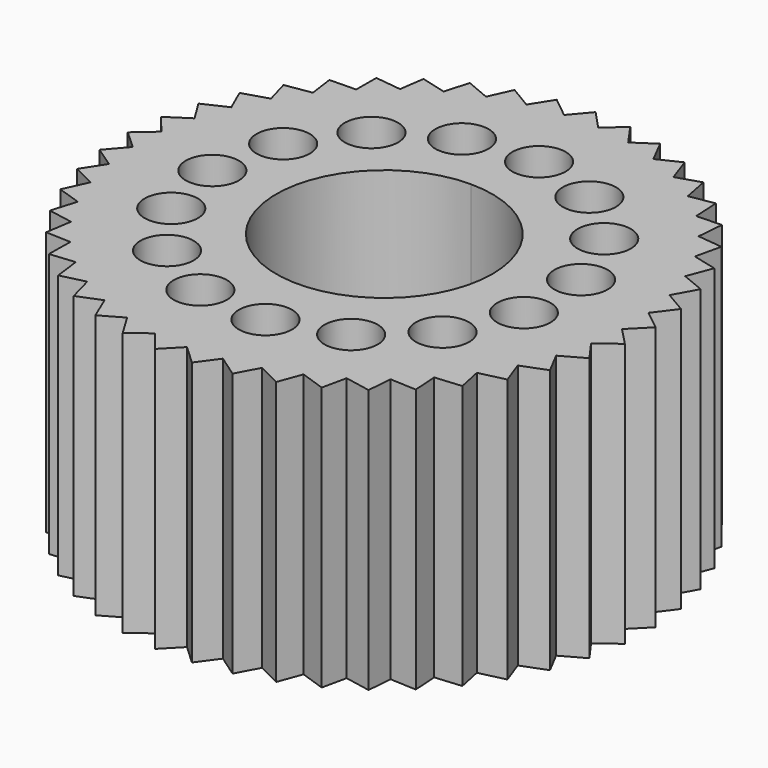
from build123d import *

# Parameters (mm, degrees)
F0_R            = 25.4
F1_DEPTH        = 25.4
F3_DEPTH        = 25.4
F6_DEPTH        = 25.4
F5_DEPTH        = 25.4
F5_COPIES_COUNT = 15


# Not quite as in the source:
# - a pattern or mirror of a feature is missing from the dataset's text; its kind, count and spacing are read off the source's solid


with BuildPart() as f1:
    # F0 (on Top) → F1 (new body)
    with BuildSketch(Plane.XY):
        Circle(F0_R)
    extrude(amount=F1_DEPTH)

    # F2 (on face) → F3 (cut)
    with BuildSketch(Plane.XY.offset(25.4)):
        with BuildLine():
            Line((-3.3733606068, -23.3670165801), (-5.2809569468, -24.8449490586))
            ThreePointArc((-5.2809569468, -24.8449490586), (-3.5349967644, -25.152808946), (-1.7718144331, -25.3381268766))
            Line((-1.7718144331, -25.3381268766), (-3.3733606068, -23.3670165801))
        make_face()
        with BuildLine():
            Line((-0.0884711356, -23.6090914373), (-1.7718144331, -25.3381268766))
            ThreePointArc((-1.7718144331, -25.3381268766), (0, -25.4), (1.7718144331, -25.3381268766))
            Line((1.7718144331, -25.3381268766), (-0.0884711356, -23.6090914373))
        make_face()
        with BuildLine():
            ThreePointArc((1.7718144331, -25.3381268766), (3.5349967644, -25.152808946), (5.2809569468, -24.8449490586))
            Line((5.2809569468, -24.8449490586), (3.1981403256, -23.3916421847))
            Line((3.1981403256, -23.3916421847), (1.7718144331, -25.3381268766))
        make_face()
        with BuildLine():
            ThreePointArc((5.2809569468, -24.8449490586), (7.0011888378, -24.4160470768), (8.6873116405, -23.868192568))
            Line((8.6873116405, -23.868192568), (6.4225036232, -22.7189012245))
            Line((6.4225036232, -22.7189012245), (5.2809569468, -24.8449490586))
        make_face()
        with BuildLine():
            ThreePointArc((8.6873116405, -23.868192568), (10.3311107341, -23.2040546241), (11.9245776948, -22.4268688586))
            Line((11.9245776948, -22.4268688586), (9.5218601932, -21.6039626944))
            Line((9.5218601932, -21.6039626944), (8.6873116405, -23.868192568))
        make_face()
        with BuildLine():
            ThreePointArc((11.9245776948, -22.4268688586), (13.4599493115, -21.5404216424), (14.9297454082, -20.5490316571))
            Line((14.9297454082, -20.5490316571), (12.4358845856, -20.0685276045))
            Line((12.4358845856, -20.0685276045), (11.9245776948, -22.4268688586))
        make_face()
        with BuildLine():
            ThreePointArc((14.9297454082, -20.5490316571), (16.326805286, -19.4575288552), (17.6443226097, -18.2712309286))
            Line((17.6443226097, -18.2712309286), (15.1078586301, -18.1424814524))
            Line((15.1078586301, -18.1424814524), (14.9297454082, -20.5490316571))
        make_face()
        with BuildLine():
            ThreePointArc((17.6443226097, -18.2712309286), (18.8758785671, -16.9959174015), (20.0154731416, -15.6378014733))
            Line((20.0154731416, -15.6378014733), (17.4857753913, -15.8633125357))
            Line((17.4857753913, -15.8633125357), (17.6443226097, -18.2712309286))
        make_face()
        with BuildLine():
            ThreePointArc((20.0154731416, -15.6378014733), (21.0575543429, -14.2034997482), (21.9970452561, -12.7))
            Line((21.9970452561, -12.7), (19.5233514242, -13.2753822847))
            Line((19.5233514242, -13.2753822847), (20.0154731416, -15.6378014733))
        make_face()
        with BuildLine():
            ThreePointArc((21.9970452561, -12.7), (22.829368776, -11.1346271284), (23.550469906, -9.5150074728))
            Line((23.550469906, -9.5150074728), (21.1809276292, -10.429061818))
            Line((21.1809276292, -10.429061818), (21.9970452561, -12.7))
        make_face()
        with BuildLine():
            ThreePointArc((23.550469906, -9.5150074728), (24.1568355139, -7.8490316571), (24.6455114474, -6.1448161482))
            Line((24.6455114474, -6.1448161482), (22.4262411709, -7.3797515259))
            Line((22.4262411709, -7.3797515259), (23.550469906, -9.5150074728))
        make_face()
        with BuildLine():
            ThreePointArc((24.6455114474, -6.1448161482), (25.0141169265, -4.4106637127), (25.2608561424, -2.655022967))
            Line((25.2608561424, -2.655022967), (23.2350534376, -4.1868027647))
            Line((23.2350534376, -4.1868027647), (24.6455114474, -6.1448161482))
        make_face()
        with BuildLine():
            ThreePointArc((25.4, 0), (25.396131457, 0.4432911235), (25.3845270063, 0.8864472162))
            Line((25.3845270063, 0.8864472162), (23.5916218186, -0.9123626502))
            Line((23.5916218186, -0.9123626502), (25.2608561424, -2.655022967))
            ThreePointArc((25.2608561424, -2.655022967), (25.3651901828, -1.3293332886), (25.4, 0))
        make_face()
        with BuildLine():
            ThreePointArc((25.3845270063, 0.8864472162), (25.2608561424, 2.655022967), (25.0141169265, 4.4106637127))
            Line((25.0141169265, 4.4106637127), (23.489006116, 2.3798355656))
            Line((23.489006116, 2.3798355656), (25.3845270063, 0.8864472162))
        make_face()
        with BuildLine():
            ThreePointArc((25.0141169265, 4.4106637127), (24.6455114474, 6.1448161482), (24.1568355139, 7.8490316571))
            Line((24.1568355139, 7.8490316571), (22.9292036277, 5.6257129891))
            Line((22.9292036277, 5.6257129891), (25.0141169265, 4.4106637127))
        make_face()
        with BuildLine():
            ThreePointArc((24.1568355139, 7.8490316571), (23.550469906, 9.5150074728), (22.829368776, 11.1346271284))
            Line((22.829368776, 11.1346271284), (21.9231102724, 8.7620923084))
            Line((21.9231102724, 8.7620923084), (24.1568355139, 7.8490316571))
        make_face()
        with BuildLine():
            ThreePointArc((22.829368776, 11.1346271284), (21.9970452561, 12.7), (21.0575543429, 14.2034997482))
            Line((21.0575543429, 14.2034997482), (20.4903085128, 11.7279274677))
            Line((20.4903085128, 11.7279274677), (22.829368776, 11.1346271284))
        make_face()
        with BuildLine():
            ThreePointArc((21.0575543429, 14.2034997482), (20.0154731416, 15.6378014733), (18.8758785671, 16.9959174015))
            Line((18.8758785671, 16.9959174015), (18.6586862054, 14.4654918592))
            Line((18.6586862054, 14.4654918592), (21.0575543429, 14.2034997482))
        make_face()
        with BuildLine():
            ThreePointArc((18.8758785671, 16.9959174015), (17.6443226097, 18.2712309286), (16.326805286, 19.4575288552))
            Line((16.326805286, 19.4575288552), (16.4638937949, 16.9215019058))
            Line((16.4638937949, 16.9215019058), (18.8758785671, 16.9959174015))
        make_face()
        with BuildLine():
            ThreePointArc((16.326805286, 19.4575288552), (14.9297454082, 20.5490316571), (13.4599493115, 21.5404216424))
            Line((13.4599493115, 21.5404216424), (13.9486504191, 19.0481541658))
            Line((13.9486504191, 19.0481541658), (16.326805286, 19.4575288552))
        make_face()
        with BuildLine():
            ThreePointArc((13.4599493115, 21.5404216424), (11.9245776948, 22.4268688586), (10.3311107341, 23.2040546241))
            Line((10.3311107341, 23.2040546241), (11.1619124293, 20.8040557719))
            Line((11.1619124293, 20.8040557719), (13.4599493115, 21.5404216424))
        make_face()
        with BuildLine():
            ThreePointArc((10.3311107341, 23.2040546241), (8.6873116405, 23.868192568), (7.0011888378, 24.4160470768))
            Line((7.0011888378, 24.4160470768), (8.1579205105, 22.1550300966))
            Line((8.1579205105, 22.1550300966), (10.3311107341, 23.2040546241))
        make_face()
        with BuildLine():
            ThreePointArc((7.0011888378, 24.4160470768), (5.2809569468, 24.8449490586), (3.5349967644, 25.152808946))
            Line((3.5349967644, 25.152808946), (4.9951439484, 23.0747819615))
            Line((4.9951439484, 23.0747819615), (7.0011888378, 24.4160470768))
        make_face()
        with BuildLine():
            ThreePointArc((3.5349967644, 25.152808946), (1.7718144331, 25.3381268766), (0, 25.4))
            Line((0, 25.4), (1.7351425913, 23.5454094427))
            Line((1.7351425913, 23.5454094427), (3.5349967644, 25.152808946))
        make_face()
        with BuildLine():
            Line((-1.5586313426, 23.5577523116), (0, 25.4))
            ThreePointArc((0, 25.4), (-1.7718144331, 25.3381268766), (-3.5349967644, 25.152808946))
            Line((-3.5349967644, 25.152808946), (-1.5586313426, 23.5577523116))
        make_face()
        with BuildLine():
            Line((-4.8220682904, 23.1115703283), (-3.5349967644, 25.152808946))
            ThreePointArc((-3.5349967644, 25.152808946), (-5.2809569468, 24.8449490586), (-7.0011888378, 24.4160470768))
            Line((-7.0011888378, 24.4160470768), (-4.8220682904, 23.1115703283))
        make_face()
        with BuildLine():
            Line((-7.9916491639, 22.2155479176), (-7.0011888378, 24.4160470768))
            ThreePointArc((-7.0011888378, 24.4160470768), (-8.6873116405, 23.868192568), (-10.3311107341, 23.2040546241))
            Line((-10.3311107341, 23.2040546241), (-7.9916491639, 22.2155479176))
        make_face()
        with BuildLine():
            Line((-11.0056816768, 20.8871251365), (-10.3311107341, 23.2040546241))
            ThreePointArc((-10.3311107341, 23.2040546241), (-11.9245776948, 22.4268688586), (-13.4599493115, 21.5404216424))
            Line((-13.4599493115, 21.5404216424), (-11.0056816768, 20.8871251365))
        make_face()
        with BuildLine():
            Line((-13.8055011147, 19.1521582233), (-13.4599493115, 21.5404216424))
            ThreePointArc((-13.4599493115, 21.5404216424), (-14.9297454082, 20.5490316571), (-16.326805286, 19.4575288552))
            Line((-16.326805286, 19.4575288552), (-13.8055011147, 19.1521582233))
        make_face()
        with BuildLine():
            Line((-16.3366121768, 17.0444163356), (-16.326805286, 19.4575288552))
            ThreePointArc((-16.326805286, 19.4575288552), (-17.6443226097, 18.2712309286), (-18.8758785671, 16.9959174015))
            Line((-18.8758785671, 16.9959174015), (-16.3366121768, 17.0444163356))
        make_face()
        with BuildLine():
            Line((-18.5497496656, 14.6049242717), (-18.8758785671, 16.9959174015))
            ThreePointArc((-18.8758785671, 16.9959174015), (-20.0154731416, 15.6378014733), (-21.0575543429, 14.2034997482))
            Line((-21.0575543429, 14.2034997482), (-18.5497496656, 14.6049242717))
        make_face()
        with BuildLine():
            Line((-20.4018373772, 11.8811639696), (-21.0575543429, 14.2034997482))
            ThreePointArc((-21.0575543429, 14.2034997482), (-21.9970452561, 12.7), (-22.829368776, 11.1346271284))
            Line((-22.829368776, 11.1346271284), (-20.4018373772, 11.8811639696))
        make_face()
        with BuildLine():
            Line((-21.856826531, 8.9261503255), (-22.829368776, 11.1346271284))
            ThreePointArc((-22.829368776, 11.1346271284), (-23.550469906, 9.5150074728), (-24.1568355139, 7.8490316571))
            Line((-24.1568355139, 7.8490316571), (-21.856826531, 8.9261503255))
        make_face()
        with BuildLine():
            Line((-22.8863974181, 5.7973993187), (-24.1568355139, 7.8490316571))
            ThreePointArc((-24.1568355139, 7.8490316571), (-24.6455114474, 6.1448161482), (-25.0141169265, 4.4106637127))
            Line((-25.0141169265, 4.4106637127), (-22.8863974181, 5.7973993187))
        make_face()
        with BuildLine():
            Line((-23.4705106123, 2.5558085286), (-25.0141169265, 4.4106637127))
            ThreePointArc((-25.0141169265, 4.4106637127), (-25.2608561424, 2.655022967), (-25.3845270063, 0.8864472162))
            Line((-25.3845270063, 0.8864472162), (-23.4705106123, 2.5558085286))
        make_face()
        with BuildLine():
            Line((-23.5977970148, -0.7355281674), (-25.3845270063, 0.8864472162))
            ThreePointArc((-25.3845270063, 0.8864472162), (-25.3845270063, -0.8864472162), (-25.2608561424, -2.655022967))
            Line((-25.2608561424, -2.655022967), (-23.5977970148, -0.7355281674))
        make_face()
        with BuildLine():
            Line((-23.2657791405, -4.0125486442), (-25.2608561424, -2.655022967))
            ThreePointArc((-25.2608561424, -2.655022967), (-25.0141169265, -4.4106637127), (-24.6455114474, -6.1448161482))
            Line((-24.6455114474, -6.1448161482), (-23.2657791405, -4.0125486442))
        make_face()
        with BuildLine():
            Line((-22.4809193397, -7.2114694259), (-24.6455114474, -6.1448161482))
            ThreePointArc((-24.6455114474, -6.1448161482), (-24.1568355139, -7.8490316571), (-23.550469906, -9.5150074728))
            Line((-23.550469906, -9.5150074728), (-22.4809193397, -7.2114694259))
        make_face()
        with BuildLine():
            Line((-21.2584940156, -10.2700271581), (-23.550469906, -9.5150074728))
            ThreePointArc((-23.550469906, -9.5150074728), (-22.829368776, -11.1346271284), (-21.9970452561, -12.7))
            Line((-21.9970452561, -12.7), (-21.2584940156, -10.2700271581))
        make_face()
        with BuildLine():
            Line((-19.6222962866, -13.1286904936), (-21.9970452561, -12.7))
            ThreePointArc((-21.9970452561, -12.7), (-21.0575543429, -14.2034997482), (-20.0154731416, -15.6378014733))
            Line((-20.0154731416, -15.6378014733), (-19.6222962866, -13.1286904936))
        make_face()
        with BuildLine():
            Line((-17.6041728805, -15.7318188024), (-20.0154731416, -15.6378014733))
            ThreePointArc((-20.0154731416, -15.6378014733), (-18.8758785671, -16.9959174015), (-17.6443226097, -18.2712309286))
            Line((-17.6443226097, -18.2712309286), (-17.6041728805, -15.7318188024))
        make_face()
        with BuildLine():
            Line((-15.2434042737, -18.0287451529), (-17.6443226097, -18.2712309286))
            ThreePointArc((-17.6443226097, -18.2712309286), (-16.326805286, -19.4575288552), (-14.9297454082, -20.5490316571))
            Line((-14.9297454082, -20.5490316571), (-15.2434042737, -18.0287451529))
        make_face()
        with BuildLine():
            Line((-12.5859401418, -19.9747624863), (-14.9297454082, -20.5490316571))
            ThreePointArc((-14.9297454082, -20.5490316571), (-13.4599493115, -21.5404216424), (-11.9245776948, -22.4268688586))
            Line((-11.9245776948, -22.4268688586), (-12.5859401418, -19.9747624863))
        make_face()
        with BuildLine():
            Line((-9.6835050014, -21.5319937889), (-11.9245776948, -22.4268688586))
            ThreePointArc((-11.9245776948, -22.4268688586), (-10.3311107341, -23.2040546241), (-8.6873116405, -23.868192568))
            Line((-8.6873116405, -23.868192568), (-9.6835050014, -21.5319937889))
        make_face()
        with BuildLine():
            Line((-6.5925914509, -22.6701293247), (-8.6873116405, -23.868192568))
            ThreePointArc((-8.6873116405, -23.868192568), (-7.0011888378, -24.4160470768), (-5.2809569468, -24.8449490586))
            Line((-5.2809569468, -24.8449490586), (-6.5925914509, -22.6701293247))
        make_face()
    extrude(amount=-F3_DEPTH, mode=Mode.SUBTRACT)

    # F2 (on face) → F6 (cut)
    with BuildSketch(Plane.XY.offset(25.4)):
        with BuildLine():
            ThreePointArc((10.3984196314, 0), (7.352793035, 7.352793035), (0, 10.3984196314))
            ThreePointArc((0, 10.3984196314), (-7.352793035, -7.352793035), (10.3984196314, 0))
        make_face()
    extrude(amount=-F6_DEPTH, mode=Mode.SUBTRACT)

    # F4 (on face) → F5 (cut, through all)
    with BuildSketch(Plane(origin=(0, 0, 0), x_dir=(1, 0, 0), z_dir=(0, 0, -1))):
        with BuildLine():
            ThreePointArc((-19.0957056503, 0), (-16.5344700217, -2.5612356286), (-13.9732343931, 0))
            Line((-13.9732343931, 0), (-19.0957056503, 0))
        make_face()
        with BuildLine():
            Line((-19.0957056503, 0), (-13.9732343931, 0))
            ThreePointArc((-13.9732343931, 0), (-16.5344700217, 2.5612356286), (-19.0957056503, 0))
        make_face()
    f5 = extrude(amount=-F5_DEPTH, mode=Mode.SUBTRACT)

    # F5_copies: F5 ×15 about axis
    f5_copies_axis = Axis((0, 0, 0), (0, 0, 1))
    for i in range(1, F5_COPIES_COUNT):
        add(f5.rotate(f5_copies_axis, i * 360 / F5_COPIES_COUNT), mode=Mode.SUBTRACT)


solid = f1.part
